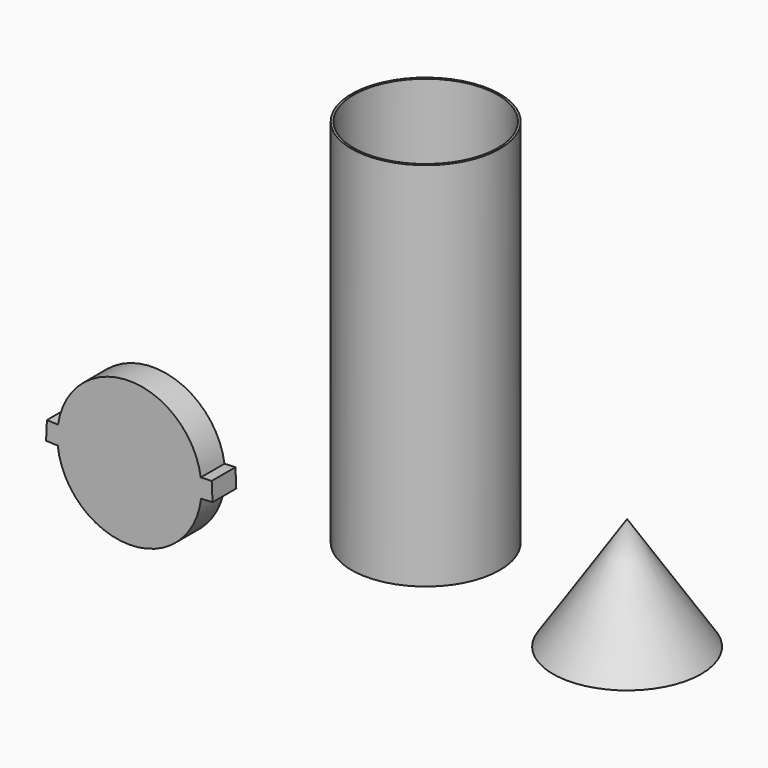
from build123d import *

# Parameters (mm, degrees)
F0_R     = 50.8
F0_R_2   = 49.3776
F1_DEPTH = 254
F4_DEPTH = 20.32
F5_W     = 12.7
F5_H     = 7.62
F6_DEPTH = 127
F8_DEPTH = 12.7


with BuildPart() as f1:
    # F0 (on Top) → F1 (new body)
    with BuildSketch(Plane.XY):
        with Locations((0, 26.6699958593)):
            Circle(F0_R)
        with Locations((0, 26.6699958593)):
            Circle(F0_R_2, mode=Mode.SUBTRACT)
    extrude(amount=F1_DEPTH)

    # F5 (on Right) → F6 (cut)
    with BuildSketch(Plane.YZ):
        with Locations((26.0630475703, 24.0578921512)):
            Rectangle(F5_W, F5_H)
    extrude(amount=-F6_DEPTH, mode=Mode.SUBTRACT)

    # F0 (on Top) → F8 (cut)
    with BuildSketch(Plane.XY):
        with Locations((0, 26.6699958593)):
            Circle(F0_R_2)
    extrude(amount=F8_DEPTH, mode=Mode.SUBTRACT)


with BuildPart() as f3:
    # F2 (on Front) → F3 (revolve)
    with BuildSketch(Plane.XZ):
        Polygon((210.0536121607, 0), (159.2536121607, 76.962), (159.2536121607, 0), (177.7075566351, 0), (191.6012279689, 0), align=None)
    revolve(axis=Axis((159.2536121607, 0, 38.481), (0, 0, -1)))


with BuildPart() as f4:
    # F2 (on Front) → F4 (new body)
    with BuildSketch(Plane.XZ):
        with BuildLine():
            Line((-238.6063388573, -5.2871476303), (-230.6097944098, -5.6449494469))
            ThreePointArc((-230.6097944098, -5.6449494469), (-181.5532885898, -49.3775999295), (-132.5014562586, -5.6397075884))
            Line((-132.5014562586, -5.6397075884), (-124.6220625717, -5.2871476303))
            Line((-124.6220625717, -5.2871476303), (-125.1897504177, 7.4001582504))
            Line((-125.1897504177, 7.4001582504), (-132.6863348709, 7.0647269208))
            ThreePointArc((-132.6863348709, 7.0647269208), (-181.5585443994, 49.3775999306), (-230.4262674829, 7.0595455428))
            Line((-230.4262674829, 7.0595455428), (-238.0386510113, 7.4001582504))
            Line((-238.0386510113, 7.4001582504), (-238.6063388573, -5.2871476303))
        make_face()
    extrude(amount=-F4_DEPTH)


solid = Compound([f1.part, f3.part, f4.part])
